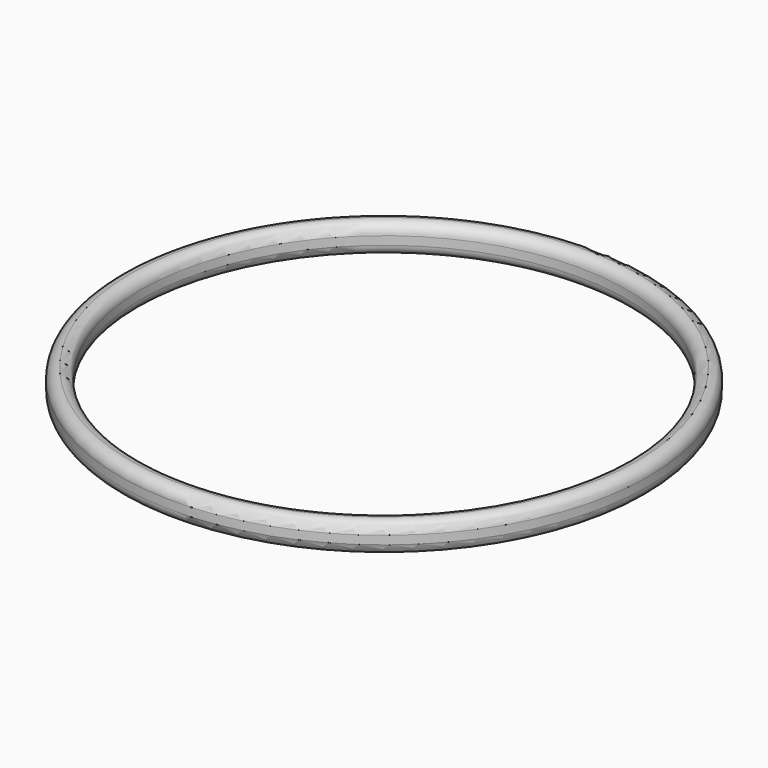
from build123d import *

# Parameters (mm, degrees)
F0_R     = 31.75
F1_DEPTH = 3.556
F3_D     = 58.42
F3_DEPTH = 5.08
F3_TIP   = 17.5511386818
F4_R     = 1.26999


# Not quite as in the source:
# - a fillet or chamfer is up to 0.001 mm smaller than in the source, because OpenCascade refuses the exact size


with BuildPart() as f1:
    # F0 (on Top) → F1 (new body)
    with BuildSketch(Plane.XY):
        Circle(F0_R)
    extrude(amount=F1_DEPTH)

    # F3
    with Locations(Plane.XY.offset(3.556)):
        with Locations((0, 0)):
            Hole(F3_D / 2, depth=F3_DEPTH)
            with Locations((0, 0, -(F3_DEPTH + F3_TIP / 2))):  # 118° drill point
                Cone(0, F3_D / 2, F3_TIP, mode=Mode.SUBTRACT)

    # F4 (radius 1.27 in the source; OpenCascade refuses exactly that, so slightly less here)
    f4_edges = [f1.edges().sort_by_distance(p)[0] for p in [
        (-31.75, 0, 0),
        (-31.75, 0, 3.556),
        (-29.21, 0, 0),
        (-29.21, 0, 3.556),
    ]]
    fillet(f4_edges, radius=F4_R)


solid = f1.part
